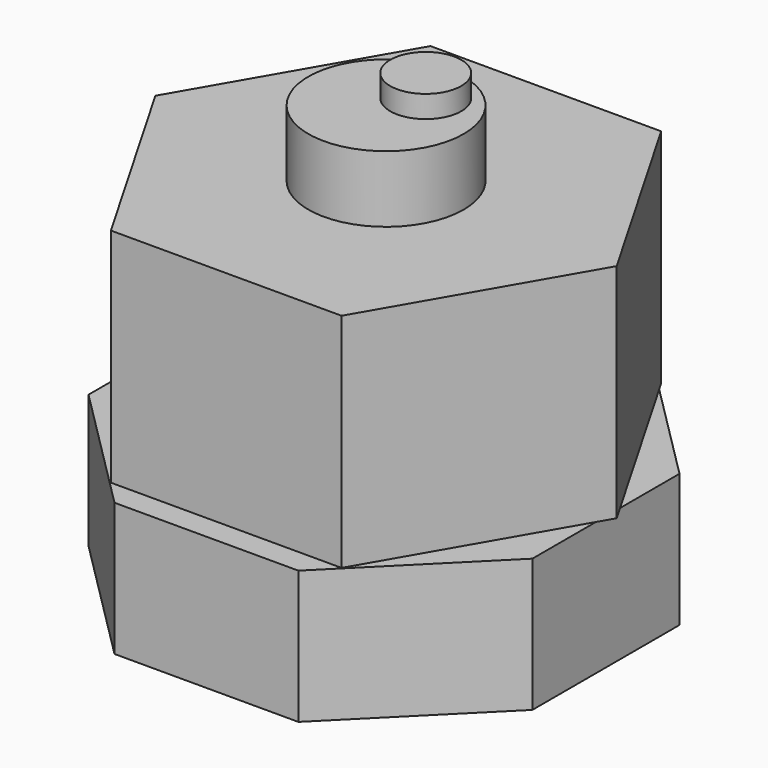
from build123d import *
from build123d import SkipClean  # not in build123d's __all__

# Parameters (mm, degrees)
F1_DEPTH  = 30
F2_R      = 17.5
F3_DEPTH  = 20
F0_R      = 17.5
F4_DEPTH  = 30
F5_R      = 17.5
F6_DEPTH  = 35
F7_DEPTH  = 30
F8_R      = 8
F9_DEPTH  = 30
F10_R     = 8
F11_DEPTH = 5
F13_DEPTH = 30
F14_R     = 8
F15_DEPTH = 30
F16_R     = 1
F17_DEPTH = 30
F18_DEPTH = 30


# Not quite as in the source:
# - after a boolean that leaves OpenCascade's solid faulty, fix() repairs it


with BuildPart() as f1:
    # F0 (on Top) → F1 (new body)
    with BuildSketch(Plane.XY):
        with BuildLine():
            ThreePointArc((7.4772695936, -0.5834718719), (7.494315244, -0.29195723), (7.5, 0))
            ThreePointArc((7.5, 0), (6.4951905284, 3.75), (3.75, 6.4951905284))
            ThreePointArc((3.75, 6.4951905284), (-0.29195723, 7.494315244), (-4.2439362602, 6.183769483))
            ThreePointArc((-4.2439362602, 6.183769483), (-0.25, -0.4330127019), (7.4772695936, -0.5834718719))
        make_face()
        with BuildLine():
            ThreePointArc((3.75, 6.4951905284), (6.4951905284, 3.75), (7.5, 0))
            ThreePointArc((7.5, 0), (7.494315244, -0.29195723), (7.4772695936, -0.5834718719))
            ThreePointArc((7.4772695936, -0.5834718719), (10.5990202492, 2.3610737393), (11.75, 6.4951905284))
            ThreePointArc((11.75, 6.4951905284), (3.5942599631, 14.4936744498), (-4.2439362602, 6.183769483))
            ThreePointArc((-4.2439362602, 6.183769483), (-0.29195723, 7.494315244), (3.75, 6.4951905284))
        make_face()
    extrude(amount=F1_DEPTH)

    # F5 (on face) → F6 (join)
    with BuildSketch(Plane.XY.offset(30)):
        Circle(F5_R)
        with BuildLine():
            ThreePointArc((-4.2439362602, 6.183769483), (7.75, 13.4233937587), (7.4772695936, -0.5834718719))
            ThreePointArc((7.4772695936, -0.5834718719), (-3.75, -6.4951905284), (-4.2439362602, 6.183769483))
        make_face(mode=Mode.SUBTRACT)
        with BuildLine():
            ThreePointArc((-4.2439362602, 6.183769483), (-3.75, -6.4951905284), (7.4772695936, -0.5834718719))
            ThreePointArc((7.4772695936, -0.5834718719), (7.75, 13.4233937587), (-4.2439362602, 6.183769483))
        make_face()
    extrude(amount=F6_DEPTH)

    # F8 (on face) → F9 (join)
    with BuildSketch(Plane.XY):
        with Locations((3.75, 6.4951905284)):
            Circle(F8_R)
    extrude(amount=-F9_DEPTH)

    # F10 (on face) → F11 (join)
    with BuildSketch(Plane.XY.offset(65)):
        with Locations((3.75, 6.4951905284)):
            Circle(F10_R)
    extrude(amount=F11_DEPTH)


with BuildPart() as f1b:
    # F0 (on Top) → F1, piece 2 (new body)
    with BuildSketch(Plane.XY):
        Polygon((25.9807621135, 45), (-25.9807621135, 45), (-51.9615242271, 0), (-25.9807621135, -45), (25.9807621135, -45), (51.9615242271, 0), align=None)
        with BuildLine():
            ThreePointArc((35, 0), (-30.3108892273, -17.4999998357), (17.5000003287, 30.3108889427))
            ThreePointArc((17.5000003287, 30.3108889427), (30.3108892273, 17.4999998357), (35, 0))
        make_face(mode=Mode.SUBTRACT)
    extrude(amount=F1_DEPTH)

    # F2 (on face) → F3 (join)
    with BuildSketch(Plane.XY.offset(30)):
        Polygon((-25.9807621135, 45), (-51.9615242271, 0), (-25.9807621135, -45), (25.9807621135, -45), (51.9615242271, 0), (25.9807621135, 45), align=None)
        Circle(F2_R, mode=Mode.SUBTRACT)
    extrude(amount=F3_DEPTH)


with BuildPart() as f4:
    # F0 (on Top) → F4 (new body)
    with BuildSketch(Plane.XY):
        with BuildLine():
            ThreePointArc((17.5000003287, 30.3108889427), (-20.0656986989, -7.2548093073), (31.25, 6.4951905284))
            ThreePointArc((31.25, 6.4951905284), (27.5656986989, 20.2451903641), (17.5000003287, 30.3108889427))
        make_face()
        Circle(F0_R, mode=Mode.SUBTRACT)
        Circle(F0_R)
        with BuildLine():
            ThreePointArc((11.75, 6.4951905284), (10.5990202492, 2.3610737393), (7.4772695936, -0.5834718719))
            ThreePointArc((7.4772695936, -0.5834718719), (-3.75, -6.4951905284), (-4.2439362602, 6.183769483))
            ThreePointArc((-4.2439362602, 6.183769483), (3.5942599631, 14.4936744498), (11.75, 6.4951905284))
        make_face(mode=Mode.SUBTRACT)
    extrude(amount=F4_DEPTH)

    # F0 (on Top) → F7 (join)
    with BuildSketch(Plane.XY):
        with BuildLine():
            ThreePointArc((17.5000003287, 30.3108889427), (-20.0656986989, -7.2548093073), (31.25, 6.4951905284))
            ThreePointArc((31.25, 6.4951905284), (27.5656986989, 20.2451903641), (17.5000003287, 30.3108889427))
        make_face()
        Circle(F0_R, mode=Mode.SUBTRACT)
        Circle(F0_R)
        with BuildLine():
            ThreePointArc((11.75, 6.4951905284), (10.5990202492, 2.3610737393), (7.4772695936, -0.5834718719))
            ThreePointArc((7.4772695936, -0.5834718719), (-3.75, -6.4951905284), (-4.2439362602, 6.183769483))
            ThreePointArc((-4.2439362602, 6.183769483), (3.5942599631, 14.4936744498), (11.75, 6.4951905284))
        make_face(mode=Mode.SUBTRACT)
        with BuildLine():
            ThreePointArc((-4.2439362602, 6.183769483), (-3.75, -6.4951905284), (7.4772695936, -0.5834718719))
            ThreePointArc((7.4772695936, -0.5834718719), (-0.25, -0.4330127019), (-4.2439362602, 6.183769483))
        make_face()
    extrude(amount=F7_DEPTH)

    # F14 (on face) → F15 (join)
    with BuildSketch(Plane.XY):
        with BuildLine():
            ThreePointArc((18.7499993484, 32.4759530181), (-22.2307619254, -8.5048097974), (33.75, 6.4951905284))
            ThreePointArc((33.75, 6.4951905284), (29.7307619254, 21.4951908542), (18.7499993484, 32.4759530181))
        make_face()
        with Locations((3.75, 6.4951905284)):
            Circle(F14_R, mode=Mode.SUBTRACT)
    with SkipClean():  # cleaning this boolean's faces spoils the solid; the shape is the same uncleaned
        extrude(amount=-F15_DEPTH)


with BuildPart() as f13:
    # F12 (on Top) → F13 (new body)
    with BuildSketch(Plane.XY):
        Polygon((50, 20.1392216345), (20.7106781187, 49.4285435158), (-20.7106781187, 49.4285435158), (-50, 20.1392216345), (-50, -21.2821346028), (-20.7106781187, -50.5714564842), (20.7106781187, -50.5714564842), (50, -21.2821346028), align=None)
        with BuildLine():
            ThreePointArc((18.7499993484, 32.4759530181), (32.4759524538, 18.7500003258), (37.5, 0))
            ThreePointArc((37.5, 0), (-32.4759524538, -18.7500003258), (18.7499993484, 32.4759530181))
        make_face(mode=Mode.SUBTRACT)
    extrude(amount=-F13_DEPTH)


with BuildPart() as f17:
    # F16 (on Top) → F17 (new body)
    with BuildSketch(Plane.XY):
        with Locations((17.5, 30.3108891325)):
            Circle(F16_R)
    extrude(amount=F17_DEPTH)


with BuildPart() as f18:
    # F16 (on Top) → F18 (new body)
    with BuildSketch(Plane.XY):
        with Locations((18.75, 32.4759526419)):
            Circle(F16_R)
    extrude(amount=-F18_DEPTH)


with BuildPart() as f1b_1:
    add(f1b.part, clean=False)

    # F19: cut F17
    add(f17.part, mode=Mode.SUBTRACT)


with BuildPart() as f4_1:
    add(f4.part, clean=False)

    # F19: cut F17
    add(f17.part, mode=Mode.SUBTRACT)

    add(f4_1.part.fix(), mode=Mode.REPLACE)

    # F20: cut F18
    add(f18.part, mode=Mode.SUBTRACT)


with BuildPart() as f13_1:
    add(f13.part, clean=False)

    # F20: cut F18
    add(f18.part, mode=Mode.SUBTRACT)


solid = Compound([f1.part, f17.part, f18.part, f1b_1.part, f4_1.part, f13_1.part])
